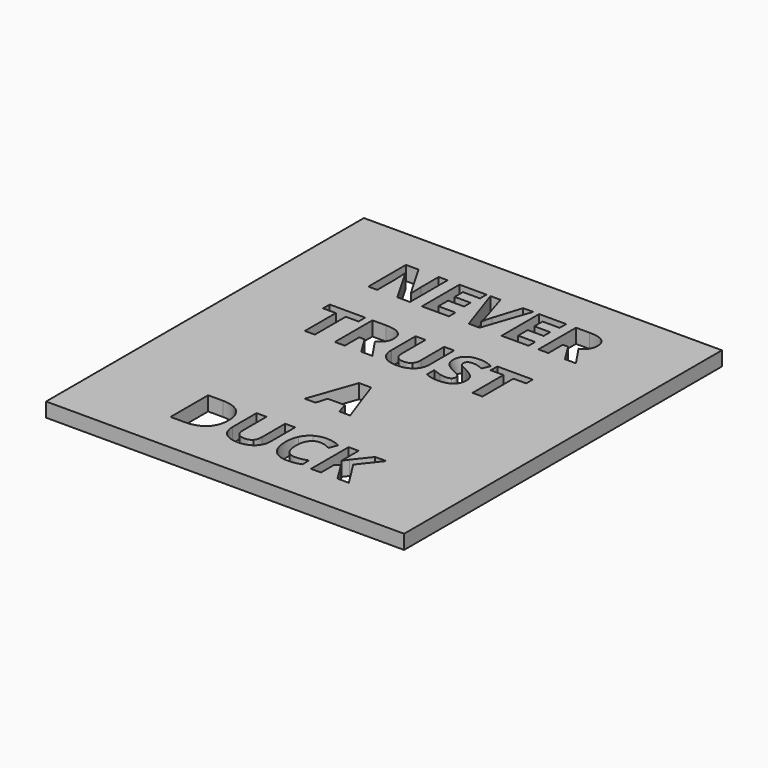
from build123d import *

# Parameters (mm, degrees)
F0_W     = 540.5047088861
F0_H     = 599.7718125582
F1_DEPTH = 21.59


with BuildPart() as f1:
    # F0 (on Top) → F1 (new body)
    with BuildSketch(Plane.XY):
        with Locations((-99.7331663966, -113.1046935916)):
            Rectangle(F0_W, F0_H)
        with BuildLine():
            add(Edge.make_bspline(
                [(-181.4957030438, -290.37537779), (-171.8814528067, -299.5469686866), (-171.8814528067, -316.0107897711)],
                knots=[0, 0, 0, 1, 1, 1], degree=2))
            add(Edge.make_bspline(
                [(-171.8814528067, -316.0107897711), (-171.8814528067, -333.53078051), (-181.8607028508, -342.8499245201)],
                knots=[0, 0, 0, 1, 1, 1], degree=2))
            add(Edge.make_bspline(
                [(-181.8607028508, -342.8499245201), (-191.839952895, -352.1690685302), (-210.6646237953, -352.1690685302)],
                knots=[0, 0, 0, 1, 1, 1], degree=2))
            Line((-210.6646237953, -352.1690685302), (-230.7629110437, -352.1690685302))
            Line((-230.7629110437, -352.1690685302), (-230.7629110437, -281.2037868935))
            Line((-230.7629110437, -281.2037868935), (-208.4901568596, -281.2037868935))
            add(Edge.make_bspline(
                [(-208.4901568596, -281.2037868935), (-191.1099532808, -281.2037868935), (-181.4957030438, -290.37537779)],
                knots=[0, 0, 0, 1, 1, 1], degree=2))
        make_face(mode=Mode.SUBTRACT)
        with BuildLine():
            Line((-114.4133980779, -281.2037868935), (-99.4095762217, -281.2037868935))
            Line((-99.4095762217, -281.2037868935), (-99.4095762217, -327.1161030498))
            add(Edge.make_bspline(
                [(-99.4095762217, -327.1161030498), (-99.4095762217, -334.9907797383), (-102.9275530855, -340.9084361847)],
                knots=[0, 0, 0, 1, 1, 1], degree=2))
            add(Edge.make_bspline(
                [(-102.9275530855, -340.9084361847), (-106.4455299493, -346.8260926311), (-113.1009519631, -349.9868356412)],
                knots=[0, 0, 0, 1, 1, 1], degree=2))
            add(Edge.make_bspline(
                [(-113.1009519631, -349.9868356412), (-119.756373977, -353.1475786513), (-128.8270074801, -353.1475786513)],
                knots=[0, 0, 0, 1, 1, 1], degree=2))
            add(Edge.make_bspline(
                [(-128.8270074801, -353.1475786513), (-142.5106172683, -353.1475786513), (-150.0824217765, -346.1271568303)],
                knots=[0, 0, 0, 1, 1, 1], degree=2))
            add(Edge.make_bspline(
                [(-150.0824217765, -346.1271568303), (-157.6542262846, -339.1067350094), (-157.6542262846, -326.9297201696)],
                knots=[0, 0, 0, 1, 1, 1], degree=2))
            Line((-157.6542262846, -326.9297201696), (-157.6542262846, -281.2037868935))
            Line((-157.6542262846, -281.2037868935), (-142.6659363351, -281.2037868935))
            Line((-142.6659363351, -281.2037868935), (-142.6659363351, -324.6465298871))
            add(Edge.make_bspline(
                [(-142.6659363351, -324.6465298871), (-142.6659363351, -332.847376616), (-139.3654061649, -336.6837575668)],
                knots=[0, 0, 0, 1, 1, 1], degree=2))
            add(Edge.make_bspline(
                [(-139.3654061649, -336.6837575668), (-136.0648759946, -340.5201385176), (-128.4387098131, -340.5201385176)],
                knots=[0, 0, 0, 1, 1, 1], degree=2))
            add(Edge.make_bspline(
                [(-128.4387098131, -340.5201385176), (-121.0610541384, -340.5201385176), (-117.7372261081, -336.6604597068)],
                knots=[0, 0, 0, 1, 1, 1], degree=2))
            add(Edge.make_bspline(
                [(-117.7372261081, -336.6604597068), (-114.4133980779, -332.8007808959), (-114.4133980779, -324.553338447)],
                knots=[0, 0, 0, 1, 1, 1], degree=2))
            Line((-114.4133980779, -324.553338447), (-114.4133980779, -281.2037868935))
        make_face(mode=Mode.SUBTRACT)
        Polygon((-67.7866142141, -216.9793527573), (-84.0019247917, -216.9793527573), (-89.1429859039, -200.0806382857), (-115.0191424385, -200.0806382857), (-120.1602035508, -216.9793527573), (-136.3755141283, -216.9793527573), (-111.3225486479, -145.7189648936), (-92.9327711347, -145.7189648936), align=None, mode=Mode.SUBTRACT)
        with BuildLine():
            add(Edge.make_bspline(
                [(-43.9762012684, -294.1185673008), (-47.9989650994, -292.7129297459), (-51.8819417703, -292.7129297459)],
                knots=[0, 0, 0, 1, 1, 1], degree=2))
            add(Edge.make_bspline(
                [(-51.8819417703, -292.7129297459), (-60.3778947261, -292.7129297459), (-65.0374667312, -299.0965433928)],
                knots=[0, 0, 0, 1, 1, 1], degree=2))
            add(Edge.make_bspline(
                [(-65.0374667312, -299.0965433928), (-69.6970387362, -305.4801570397), (-69.6970387362, -316.8805765454)],
                knots=[0, 0, 0, 1, 1, 1], degree=2))
            add(Edge.make_bspline(
                [(-69.6970387362, -316.8805765454), (-69.6970387362, -340.6133299577), (-51.8819417703, -340.6133299577)],
                knots=[0, 0, 0, 1, 1, 1], degree=2))
            add(Edge.make_bspline(
                [(-51.8819417703, -340.6133299577), (-44.4110946555, -340.6133299577), (-33.787270484, -336.8856723537)],
                knots=[0, 0, 0, 1, 1, 1], degree=2))
            Line((-33.787270484, -336.8856723537), (-33.787270484, -349.4975805806))
            add(Edge.make_bspline(
                [(-33.787270484, -349.4975805806), (-42.5162020401, -353.1475786513), (-53.2953452785, -353.1475786513)],
                knots=[0, 0, 0, 1, 1, 1], degree=2))
            add(Edge.make_bspline(
                [(-53.2953452785, -353.1475786513), (-68.7806562419, -353.1475786513), (-76.9815029707, -343.7507751078)],
                knots=[0, 0, 0, 1, 1, 1], degree=2))
            add(Edge.make_bspline(
                [(-76.9815029707, -343.7507751078), (-85.1823496996, -334.3539715643), (-85.1823496996, -316.7873851053)],
                knots=[0, 0, 0, 1, 1, 1], degree=2))
            add(Edge.make_bspline(
                [(-85.1823496996, -316.7873851053), (-85.1823496996, -305.71313564), (-81.1518199152, -297.3880336576)],
                knots=[0, 0, 0, 1, 1, 1], degree=2))
            add(Edge.make_bspline(
                [(-81.1518199152, -297.3880336576), (-77.1212901309, -289.0629316753), (-69.5727834827, -284.6285723172)],
                knots=[0, 0, 0, 1, 1, 1], degree=2))
            add(Edge.make_bspline(
                [(-69.5727834827, -284.6285723172), (-62.0242768346, -280.194212959), (-51.8819417703, -280.194212959)],
                knots=[0, 0, 0, 1, 1, 1], degree=2))
            add(Edge.make_bspline(
                [(-51.8819417703, -280.194212959), (-41.5532238258, -280.194212959), (-31.1157825345, -285.1799550044)],
                knots=[0, 0, 0, 1, 1, 1], degree=2))
            Line((-31.1157825345, -285.1799550044), (-35.9617374197, -297.419097471))
            add(Edge.make_bspline(
                [(-35.9617374197, -297.419097471), (-39.9534374374, -295.5242048556), (-43.9762012684, -294.1185673008)],
                knots=[0, 0, 0, 1, 1, 1], degree=2))
        make_face(mode=Mode.SUBTRACT)
        Polygon((13.4452577404, -312.6093022074), (38.389499874, -352.1690685302), (21.3044025222, -352.1690685302), (2.7127102221, -322.2701481645), (-3.6398396114, -326.8365287295), (-3.6398396114, -352.1690685302), (-18.6902571877, -352.1690685302), (-18.6902571877, -281.2037868935), (-3.6398396114, -281.2037868935), (-3.6398396114, -313.6810037686), (2.277816835, -305.3248379729), (21.5063173091, -281.2037868935), (38.2031169938, -281.2037868935), align=None, mode=Mode.SUBTRACT)
        Polygon((-229.2097203754, -23.3430721346), (-229.2097203754, -81.7896369845), (-244.2601379516, -81.7896369845), (-244.2601379516, -23.3430721346), (-263.5352341458, -23.3430721346), (-263.5352341458, -10.8243553477), (-209.9501560879, -10.8243553477), (-209.9501560879, -23.3430721346), align=None, mode=Mode.SUBTRACT)
        with BuildLine():
            Line((-175.9818761711, -54.5622045684), (-183.9808081131, -54.5622045684))
            Line((-183.9808081131, -54.5622045684), (-183.9808081131, -81.7896369845))
            Line((-183.9808081131, -81.7896369845), (-199.0312256894, -81.7896369845))
            Line((-199.0312256894, -81.7896369845), (-199.0312256894, -10.8243553477))
            Line((-199.0312256894, -10.8243553477), (-178.3582578937, -10.8243553477))
            add(Edge.make_bspline(
                [(-178.3582578937, -10.8243553477), (-163.8825208647, -10.8243553477), (-156.9475245306, -16.0896717134)],
                knots=[0, 0, 0, 1, 1, 1], degree=2))
            add(Edge.make_bspline(
                [(-156.9475245306, -16.0896717134), (-150.0125281964, -21.3549880791), (-150.0125281964, -32.0875355974)],
                knots=[0, 0, 0, 1, 1, 1], degree=2))
            add(Edge.make_bspline(
                [(-150.0125281964, -32.0875355974), (-150.0125281964, -38.3468939908), (-153.4528455268, -43.2239126894)],
                knots=[0, 0, 0, 1, 1, 1], degree=2))
            add(Edge.make_bspline(
                [(-153.4528455268, -43.2239126894), (-156.8931628572, -48.100931388), (-163.2146488773, -50.8656107777)],
                knots=[0, 0, 0, 1, 1, 1], degree=2))
            add(Edge.make_bspline(
                [(-163.2146488773, -50.8656107777), (-147.18572118, -74.8002789769), (-142.3397662948, -81.7896369845)],
                knots=[0, 0, 0, 1, 1, 1], degree=2))
            Line((-142.3397662948, -81.7896369845), (-159.0365659795, -81.7896369845))
            Line((-159.0365659795, -81.7896369845), (-175.9818761711, -54.5622045684))
        make_face(mode=Mode.SUBTRACT)
        with BuildLine():
            Line((-90.6495808522, -10.8243553477), (-75.645758996, -10.8243553477))
            Line((-75.645758996, -10.8243553477), (-75.645758996, -56.736671504))
            add(Edge.make_bspline(
                [(-75.645758996, -56.736671504), (-75.645758996, -64.6113481926), (-79.1637358598, -70.529004639)],
                knots=[0, 0, 0, 1, 1, 1], degree=2))
            add(Edge.make_bspline(
                [(-79.1637358598, -70.529004639), (-82.6817127236, -76.4466610854), (-89.3371347374, -79.6074040954)],
                knots=[0, 0, 0, 1, 1, 1], degree=2))
            add(Edge.make_bspline(
                [(-89.3371347374, -79.6074040954), (-95.9925567513, -82.7681471055), (-105.0631902544, -82.7681471055)],
                knots=[0, 0, 0, 1, 1, 1], degree=2))
            add(Edge.make_bspline(
                [(-105.0631902544, -82.7681471055), (-118.7468000426, -82.7681471055), (-126.3186045508, -75.7477252846)],
                knots=[0, 0, 0, 1, 1, 1], degree=2))
            add(Edge.make_bspline(
                [(-126.3186045508, -75.7477252846), (-133.8904090589, -68.7273034637), (-133.8904090589, -56.5502886238)],
                knots=[0, 0, 0, 1, 1, 1], degree=2))
            Line((-133.8904090589, -56.5502886238), (-133.8904090589, -10.8243553477))
            Line((-133.8904090589, -10.8243553477), (-118.9021191094, -10.8243553477))
            Line((-118.9021191094, -10.8243553477), (-118.9021191094, -54.2670983414))
            add(Edge.make_bspline(
                [(-118.9021191094, -54.2670983414), (-118.9021191094, -62.4679450702), (-115.6015889392, -66.3043260211)],
                knots=[0, 0, 0, 1, 1, 1], degree=2))
            add(Edge.make_bspline(
                [(-115.6015889392, -66.3043260211), (-112.3010587689, -70.1407069719), (-104.6748925874, -70.1407069719)],
                knots=[0, 0, 0, 1, 1, 1], degree=2))
            add(Edge.make_bspline(
                [(-104.6748925874, -70.1407069719), (-97.2972369127, -70.1407069719), (-93.9734088824, -66.281028161)],
                knots=[0, 0, 0, 1, 1, 1], degree=2))
            add(Edge.make_bspline(
                [(-93.9734088824, -66.281028161), (-90.6495808522, -62.4213493502), (-90.6495808522, -54.1739069013)],
                knots=[0, 0, 0, 1, 1, 1], degree=2))
            Line((-90.6495808522, -54.1739069013), (-90.6495808522, -10.8243553477))
        make_face(mode=Mode.SUBTRACT)
        with BuildLine():
            Line((-193.6416540702, 124.3653604251), (-193.6416540702, 53.4000787884))
            Line((-193.6416540702, 53.4000787884), (-212.7614311976, 53.4000787884))
            Line((-212.7614311976, 53.4000787884), (-243.6388616843, 107.0783482864))
            Line((-243.6388616843, 107.0783482864), (-244.0737550714, 107.0783482864))
            add(Edge.make_bspline(
                [(-244.0737550714, 107.0783482864), (-243.1418406704, 92.8666536711), (-243.1418406704, 86.7936781578)],
                knots=[0, 0, 0, 1, 1, 1], degree=2))
            Line((-243.1418406704, 86.7936781578), (-243.1418406704, 53.4000787884))
            Line((-243.1418406704, 53.4000787884), (-256.5924718583, 53.4000787884))
            Line((-256.5924718583, 53.4000787884), (-256.5924718583, 124.3653604251))
            Line((-256.5924718583, 124.3653604251), (-237.6124818911, 124.3653604251))
            Line((-237.6124818911, 124.3653604251), (-206.7971790311, 71.2151757543))
            Line((-206.7971790311, 71.2151757543), (-206.4554770841, 71.2151757543))
            add(Edge.make_bspline(
                [(-206.4554770841, 71.2151757543), (-207.1854766982, 85.0541046093), (-207.1854766982, 90.7698462688)],
                knots=[0, 0, 0, 1, 1, 1], degree=2))
            Line((-207.1854766982, 90.7698462688), (-207.1854766982, 124.3653604251))
            Line((-207.1854766982, 124.3653604251), (-193.6416540702, 124.3653604251))
        make_face(mode=Mode.SUBTRACT)
        Polygon((-134.9155149001, 65.8256041352), (-134.9155149001, 53.4000787884), (-175.7799613843, 53.4000787884), (-175.7799613843, 124.3653604251), (-134.9155149001, 124.3653604251), (-134.9155149001, 112.0330265185), (-160.729543808, 112.0330265185), (-160.729543808, 96.454524115), (-136.7016841687, 96.454524115), (-136.7016841687, 84.1221902083), (-160.729543808, 84.1221902083), (-160.729543808, 65.8256041352), align=None, mode=Mode.SUBTRACT)
        with BuildLine():
            add(Edge.make_bspline(
                [(-20.0648309292, -50.3608238105), (-16.3760030919, -55.1368851156), (-16.3760030919, -62.0796474032)],
                knots=[0, 0, 0, 1, 1, 1], degree=2))
            add(Edge.make_bspline(
                [(-16.3760030919, -62.0796474032), (-16.3760030919, -71.6938976402), (-23.2954675193, -77.2310223729)],
                knots=[0, 0, 0, 1, 1, 1], degree=2))
            add(Edge.make_bspline(
                [(-23.2954675193, -77.2310223729), (-30.2149319468, -82.7681471055), (-42.5317339468, -82.7681471055)],
                knots=[0, 0, 0, 1, 1, 1], degree=2))
            add(Edge.make_bspline(
                [(-42.5317339468, -82.7681471055), (-53.9010896391, -82.7681471055), (-62.6300211952, -78.4813408609)],
                knots=[0, 0, 0, 1, 1, 1], degree=2))
            Line((-62.6300211952, -78.4813408609), (-62.6300211952, -64.5026248458))
            add(Edge.make_bspline(
                [(-62.6300211952, -64.5026248458), (-55.4542803075, -67.7177295292), (-50.4763042154, -69.0224096907)],
                knots=[0, 0, 0, 1, 1, 1], degree=2))
            add(Edge.make_bspline(
                [(-50.4763042154, -69.0224096907), (-45.4983281234, -70.3270898521), (-41.3668409456, -70.3270898521)],
                knots=[0, 0, 0, 1, 1, 1], degree=2))
            add(Edge.make_bspline(
                [(-41.3668409456, -70.3270898521), (-36.4276946202, -70.3270898521), (-33.7795045307, -68.43996319)],
                knots=[0, 0, 0, 1, 1, 1], degree=2))
            add(Edge.make_bspline(
                [(-33.7795045307, -68.43996319), (-31.1313144412, -66.552836528), (-31.1313144412, -62.8096470173)],
                knots=[0, 0, 0, 1, 1, 1], degree=2))
            add(Edge.make_bspline(
                [(-31.1313144412, -62.8096470173), (-31.1313144412, -60.7283715217), (-32.2962074424, -59.0975213199)],
                knots=[0, 0, 0, 1, 1, 1], degree=2))
            add(Edge.make_bspline(
                [(-32.2962074424, -59.0975213199), (-33.4611004437, -57.4666711182), (-35.7209928661, -55.9678421232)],
                knots=[0, 0, 0, 1, 1, 1], degree=2))
            add(Edge.make_bspline(
                [(-35.7209928661, -55.9678421232), (-37.9808852886, -54.4690131283), (-44.9236475761, -51.1607170047)],
                knots=[0, 0, 0, 1, 1, 1], degree=2))
            add(Edge.make_bspline(
                [(-44.9236475761, -51.1607170047), (-51.4159845698, -48.100931388), (-54.6699190199, -45.2896562783)],
                knots=[0, 0, 0, 1, 1, 1], degree=2))
            add(Edge.make_bspline(
                [(-54.6699190199, -45.2896562783), (-57.9238534701, -42.4783811686), (-59.8653418056, -38.7351916579)],
                knots=[0, 0, 0, 1, 1, 1], degree=2))
            add(Edge.make_bspline(
                [(-59.8653418056, -38.7351916579), (-61.806830141, -34.9920021472), (-61.806830141, -30.0062601018)],
                knots=[0, 0, 0, 1, 1, 1], degree=2))
            add(Edge.make_bspline(
                [(-61.806830141, -30.0062601018), (-61.806830141, -20.5783927449), (-55.4232164941, -15.1965870791)],
                knots=[0, 0, 0, 1, 1, 1], degree=2))
            add(Edge.make_bspline(
                [(-55.4232164941, -15.1965870791), (-49.0396028472, -9.8147814133), (-37.7789705017, -9.8147814133)],
                knots=[0, 0, 0, 1, 1, 1], degree=2))
            add(Edge.make_bspline(
                [(-37.7789705017, -9.8147814133), (-32.2496117224, -9.8147814133), (-27.2250399103, -11.1194615747)],
                knots=[0, 0, 0, 1, 1, 1], degree=2))
            add(Edge.make_bspline(
                [(-27.2250399103, -11.1194615747), (-22.2004680982, -12.4241417361), (-16.7177050389, -14.8005234587)],
                knots=[0, 0, 0, 1, 1, 1], degree=2))
            Line((-16.7177050389, -14.8005234587), (-21.5636599241, -26.511581098))
            add(Edge.make_bspline(
                [(-21.5636599241, -26.511581098), (-27.2483377703, -24.1817950955), (-30.9604634676, -23.2576466478)],
                knots=[0, 0, 0, 1, 1, 1], degree=2))
            add(Edge.make_bspline(
                [(-30.9604634676, -23.2576466478), (-34.672589165, -22.3334982002), (-38.2604596089, -22.3334982002)],
                knots=[0, 0, 0, 1, 1, 1], degree=2))
            add(Edge.make_bspline(
                [(-38.2604596089, -22.3334982002), (-42.5317339468, -22.3334982002), (-44.8149242293, -24.3215822557)],
                knots=[0, 0, 0, 1, 1, 1], degree=2))
            add(Edge.make_bspline(
                [(-44.8149242293, -24.3215822557), (-47.0981145118, -26.3096663111), (-47.0981145118, -29.5092390879)],
                knots=[0, 0, 0, 1, 1, 1], degree=2))
            add(Edge.make_bspline(
                [(-47.0981145118, -29.5092390879), (-47.0981145118, -31.4973231434), (-46.1739660641, -32.9806202317)],
                knots=[0, 0, 0, 1, 1, 1], degree=2))
            add(Edge.make_bspline(
                [(-46.1739660641, -32.9806202317), (-45.2498176164, -34.46391732), (-43.2384357009, -35.8462570148)],
                knots=[0, 0, 0, 1, 1, 1], degree=2))
            add(Edge.make_bspline(
                [(-43.2384357009, -35.8462570148), (-41.2270537854, -37.2285967096), (-33.7096109506, -40.8164671535)],
                knots=[0, 0, 0, 1, 1, 1], degree=2))
            add(Edge.make_bspline(
                [(-33.7096109506, -40.8164671535), (-23.7536587665, -45.5847625053), (-20.0648309292, -50.3608238105)],
                knots=[0, 0, 0, 1, 1, 1], degree=2))
        make_face(mode=Mode.SUBTRACT)
        Polygon((23.867167125, -23.3430721346), (23.867167125, -81.7896369845), (8.8167495487, -81.7896369845), (8.8167495487, -23.3430721346), (-10.4583466455, -23.3430721346), (-10.4583466455, -10.8243553477), (43.1267314125, -10.8243553477), (43.1267314125, -23.3430721346), align=None, mode=Mode.SUBTRACT)
        with BuildLine():
            Line((-93.0725582948, 82.1341061528), (-79.6374590136, 124.3653604251))
            Line((-79.6374590136, 124.3653604251), (-64.4472542772, 124.3653604251))
            Line((-64.4472542772, 124.3653604251), (-88.5683053566, 53.4000787884))
            Line((-88.5683053566, 53.4000787884), (-104.9699988143, 53.4000787884))
            Line((-104.9699988143, 53.4000787884), (-129.0444541737, 124.3653604251))
            Line((-129.0444541737, 124.3653604251), (-113.8542494373, 124.3653604251))
            Line((-113.8542494373, 124.3653604251), (-100.4968096895, 82.1341061528))
            add(Edge.make_bspline(
                [(-100.4968096895, 82.1341061528), (-99.394044315, 78.3909166421), (-98.1980875004, 73.4207065034)],
                knots=[0, 0, 0, 1, 1, 1], degree=2))
            add(Edge.make_bspline(
                [(-98.1980875004, 73.4207065034), (-97.0021306857, 68.4504963647), (-96.7225563654, 66.5090080292)],
                knots=[0, 0, 0, 1, 1, 1], degree=2))
            add(Edge.make_bspline(
                [(-96.7225563654, 66.5090080292), (-96.1789396315, 70.9666652474), (-93.0725582948, 82.1341061528)],
                knots=[0, 0, 0, 1, 1, 1], degree=2))
        make_face(mode=Mode.SUBTRACT)
        Polygon((-14.65196145, 65.8256041352), (-14.65196145, 53.4000787884), (-55.5164079342, 53.4000787884), (-55.5164079342, 124.3653604251), (-14.65196145, 124.3653604251), (-14.65196145, 112.0330265185), (-40.4659903579, 112.0330265185), (-40.4659903579, 96.454524115), (-16.4381307186, 96.454524115), (-16.4381307186, 84.1221902083), (-40.4659903579, 84.1221902083), (-40.4659903579, 65.8256041352), align=None, mode=Mode.SUBTRACT)
        with BuildLine():
            Line((23.1992951376, 80.6275112045), (15.2003631956, 80.6275112045))
            Line((15.2003631956, 80.6275112045), (15.2003631956, 53.4000787884))
            Line((15.2003631956, 53.4000787884), (0.1499456193, 53.4000787884))
            Line((0.1499456193, 53.4000787884), (0.1499456193, 124.3653604251))
            Line((0.1499456193, 124.3653604251), (20.822913415, 124.3653604251))
            add(Edge.make_bspline(
                [(20.822913415, 124.3653604251), (35.298650444, 124.3653604251), (42.2336467782, 119.1000440595)],
                knots=[0, 0, 0, 1, 1, 1], degree=2))
            add(Edge.make_bspline(
                [(42.2336467782, 119.1000440595), (49.1686431124, 113.8347276938), (49.1686431124, 103.1021801755)],
                knots=[0, 0, 0, 1, 1, 1], degree=2))
            add(Edge.make_bspline(
                [(49.1686431124, 103.1021801755), (49.1686431124, 96.842821782), (45.728325782, 91.9658030834)],
                knots=[0, 0, 0, 1, 1, 1], degree=2))
            add(Edge.make_bspline(
                [(45.728325782, 91.9658030834), (42.2880084516, 87.0887843848), (35.9665224314, 84.3241049952)],
                knots=[0, 0, 0, 1, 1, 1], degree=2))
            add(Edge.make_bspline(
                [(35.9665224314, 84.3241049952), (51.9954501287, 60.389436796), (56.841405014, 53.4000787884)],
                knots=[0, 0, 0, 1, 1, 1], degree=2))
            Line((56.841405014, 53.4000787884), (40.1446053293, 53.4000787884))
            Line((40.1446053293, 53.4000787884), (23.1992951376, 80.6275112045))
        make_face(mode=Mode.SUBTRACT)
    extrude(amount=F1_DEPTH)


solid = f1.part
